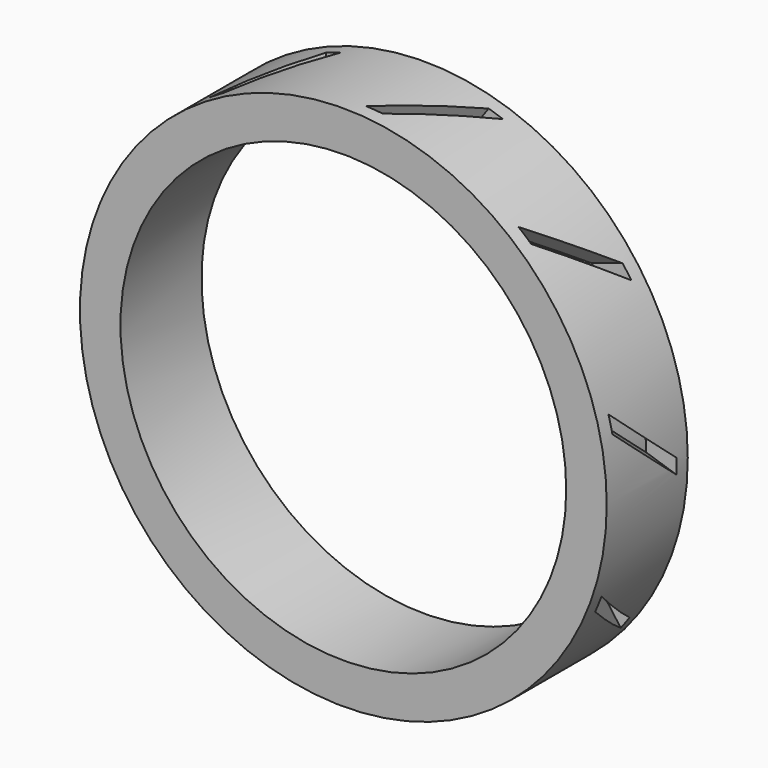
from build123d import *

# Parameters (mm, degrees)
F0_R            = 13
F0_R_2          = 11
F1_DEPTH        = 5
F3_DEPTH        = 25
F3_COPIES_COUNT = 10
F4_R            = 11.5
F4_R_2          = 11
F5_DEPTH        = 5


# Not quite as in the source:
# - a pattern or mirror of a feature is missing from the dataset's text; its kind, count and spacing are read off the source's solid


with BuildPart() as f1:
    # F0 (on Front) → F1 (new body)
    with BuildSketch(Plane.XZ):
        Circle(F0_R)
        Circle(F0_R_2, mode=Mode.SUBTRACT)
    extrude(amount=F1_DEPTH)

    # F2 (on Top) → F3 (cut)
    with BuildSketch(Plane.XY):
        Polygon((-4.2959866114, -0.7), (-7.1845799685, -4.3), (-6.4808833413, -4.3), (-3.5922899842, -0.7), align=None)
    f3 = extrude(amount=F3_DEPTH, mode=Mode.SUBTRACT)

    # F3_copies: F3 ×10 about axis
    f3_copies_axis = Axis((0, 0, 0), (0, 1, 0))
    for i in range(1, F3_COPIES_COUNT):
        add(f3.rotate(f3_copies_axis, i * 360 / F3_COPIES_COUNT), mode=Mode.SUBTRACT)

    # F4 (on Front) → F5 (join)
    with BuildSketch(Plane.XZ):
        Circle(F4_R)
        Circle(F4_R_2, mode=Mode.SUBTRACT)
    extrude(amount=F5_DEPTH)


solid = f1.part
